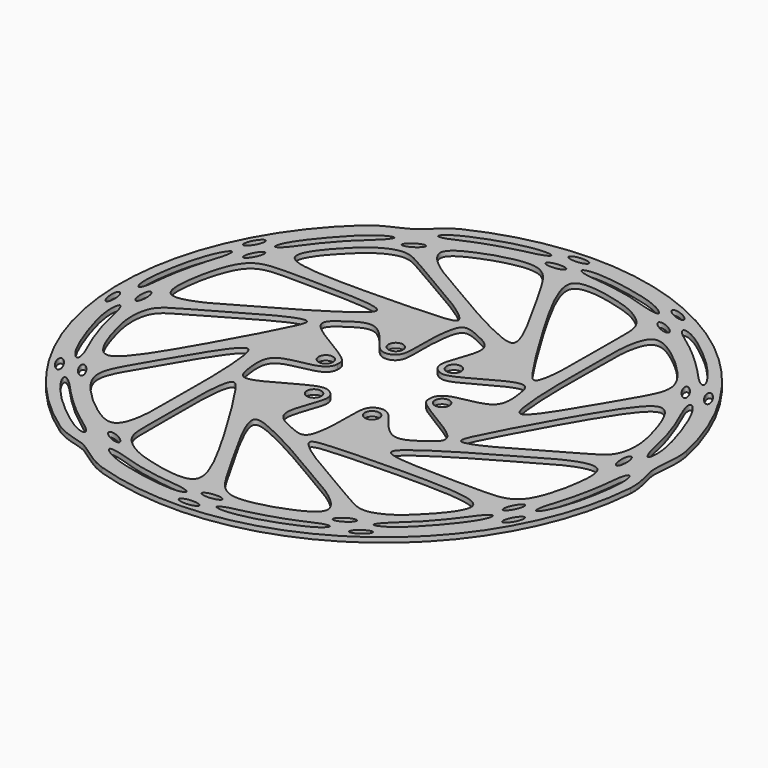
from build123d import *

# Parameters (mm, degrees)
F0_R             = 100
F1_DEPTH         = 1.85
F2_R             = 2.743128254
F3_DEPTH         = 1.851
F3_COPIES_COUNT  = 6
F7_DEPTH         = 1.8510001
F7_COPIES_COUNT  = 3
F10_DEPTH        = 1.8510001
F10_COPIES_COUNT = 2


# Not quite as in the source:
# - a pattern or mirror of a feature is missing from the dataset's text; its kind, count and spacing are read off the source's solid


with BuildPart() as f1:
    # F0 (on Top) → F1 (new body)
    with BuildSketch(Plane.XY):
        Circle(F0_R)
    extrude(amount=F1_DEPTH)

    # F2 (on Top) → F3 (cut, through all)
    with BuildSketch(Plane.XY):
        with BuildLine():
            add(Edge.make_bspline(
                [(-19.3818919361, 84.770321846), (-15.8888721091, 85.5119795187), (-7.6996501995, 86.6691177995), (-1.2711069947, 76.0041983595), (2.7590544213, 68.8211609673), (14.2848097306, 48.826735121), (15.6555298575, 41.0029385401), (4.0306774131, 45.832846657), (-11.3442409562, 54.3632933665), (-25.1795732316, 62.8245536026), (-31.577920473, 66.1201997026), (-42.6321499163, 75.6247304734), (-28.620182769, 82.2286800508), (-22.8365351394, 84.0368125145), (-19.3818919361, 84.770321846)],
                knots=[0, 0, 0, 0, 0.0806437638, 0.1605805509, 0.2363933489, 0.3555478125, 0.4090968647, 0.4834244698, 0.5923152663, 0.6895970753, 0.7594857624, 0.8380620694, 0.9202422418, 1, 1, 1, 1], degree=3))
        make_face()
        with BuildLine():
            add(Edge.make_bspline(
                [(4.0786904283, 83.0234959722), (4.8408661308, 85.0940211581), (10.9812602111, 85.7206275438), (19.6535574621, 83.7725691497), (28.668941965, 81.3282055643), (36.9257742239, 75.2245847174), (36.9680314736, 65.9345839836), (36.8019909238, 45.080539991), (36.8744568041, 36.732354482), (35.337710167, 25.8934041706), (29.5967546476, 32.9556866993), (17.5290674718, 52.9370163353), (11.4660357229, 63.1418800906), (2.7822748423, 79.5016556493), (4.0786904283, 83.0234959722)],
                knots=[0, 0, 0, 0, 0.0635478904, 0.1391827355, 0.2151092654, 0.2891479476, 0.3630886814, 0.4747583724, 0.5526009533, 0.6195279395, 0.6767941119, 0.7963800874, 0.8919088141, 1, 1, 1, 1], degree=3))
        make_face()
        with Locations((11.2100625411, 19.0960504115)):
            Circle(F2_R)
        with BuildLine():
            add(Edge.make_bspline(
                [(1.3292516815, 91.8782353401), (1.2925002073, 92.3354583441), (4.9372757242, 93.8495882438), (20.9611120073, 91.4975725839), (33.039082784, 87.9708444738), (37.8500908983, 83.7397445096), (31.1774053281, 84.75909445), (24.9839859282, 87.3881882236), (11.578213695, 89.906480861), (4.1885603815, 90.1973514145), (1.3641017607, 91.4446674832), (1.3292516815, 91.8782353401)],
                knots=[0, 0, 0, 0, 0.069104069, 0.2382448936, 0.392001905, 0.4676969543, 0.5517462119, 0.6661598603, 0.8182820791, 0.9344711381, 1, 1, 1, 1], degree=3))
        make_face()
        with BuildLine():
            add(Edge.make_bspline(
                [(-2.7077326085, 89.5969420671), (-2.8745052619, 91.7024450684), (-8.261381892, 90.2164050531), (-13.6482585222, 88.7303650379), (-8.0946092387, 88.1109020519), (-2.5409599552, 87.4914390659), (-2.7077326085, 89.5969420671)],
                knots=[0, 0, 0, 2.0943951024, 2.0943951024, 4.1887902048, 4.1887902048, 6.2831853072, 6.2831853072, 6.2831853072], degree=2, weights=[1, 0.5, 1, 0.5, 1, 0.5, 1]))
        make_face()
        with BuildLine():
            add(Edge.make_bspline(
                [(0.2530701458, 96.746198833), (0.1434808405, 98.981842031), (-5.3261488772, 97.5932179043), (-10.7957785949, 96.2045937777), (-5.2165595719, 95.3575747063), (0.3626594512, 94.510555635), (0.2530701458, 96.746198833)],
                knots=[0, 0, 0, 2.0943951024, 2.0943951024, 4.1887902048, 4.1887902048, 6.2831853072, 6.2831853072, 6.2831853072], degree=2, weights=[1, 0.5, 1, 0.5, 1, 0.5, 1]))
        make_face()
        with BuildLine():
            add(Edge.make_bspline(
                [(-45.5902777612, 82.5898870826), (-45.8140727222, 82.9738085349), (-43.585623242, 85.7456500755), (-33.1460813636, 90.1844826755), (-22.9095160971, 93.5693996934), (-13.6129666728, 94.789503836), (-10.8334910775, 93.6639122431), (-14.5180403097, 91.7933261946), (-21.5013009013, 90.6303087594), (-35.2407786326, 86.3505494796), (-42.3849200633, 82.5115902384), (-45.3821119555, 82.2327775296), (-45.5902777612, 82.5898870826)],
                knots=[0, 0, 0, 0, 0.065019585, 0.198537651, 0.3338114005, 0.4526335757, 0.5018406824, 0.5658849331, 0.6740049001, 0.8245613986, 0.9395211838, 1, 1, 1, 1], degree=3))
        make_face()
    f3 = extrude(amount=F3_DEPTH, mode=Mode.SUBTRACT)

    # F3_copies: F3 ×6 about axis
    f3_copies_axis = Axis((0, 0, 0), (0, 0, 1))
    for i in range(1, F3_COPIES_COUNT):
        add(f3.rotate(f3_copies_axis, i * 360 / F3_COPIES_COUNT), mode=Mode.SUBTRACT)

    # F5 (on Top) → F7 (cut, through all)
    with BuildSketch(Plane.XY):
        with BuildLine():
            add(Edge.make_bspline(
                [(44.7057709098, 85.9585851431), (45.5545956472, 87.8521204143), (40.2434163829, 89.0959687605), (34.9322371185, 90.3398171067), (39.3945916454, 87.2024334893), (43.8569461723, 84.0650498719), (44.7057709098, 85.9585851431)],
                knots=[0, 0, 0, 2.0943951024, 2.0943951024, 4.1887902048, 4.1887902048, 6.2831853072, 6.2831853072, 6.2831853072], degree=2, weights=[1, 0.5, 1, 0.5, 1, 0.5, 1]))
        make_face()
        with BuildLine():
            add(Edge.make_bspline(
                [(46.2925173342, 76.8029242754), (47.3216432051, 78.7262145228), (42.0045682647, 80.3343268011), (36.6874933243, 81.9424390793), (40.9754423938, 78.4110365536), (45.2633914634, 74.879634028), (46.2925173342, 76.8029242754)],
                knots=[0, 0, 0, 2.0943951024, 2.0943951024, 4.1887902048, 4.1887902048, 6.2831853072, 6.2831853072, 6.2831853072], degree=2, weights=[1, 0.5, 1, 0.5, 1, 0.5, 1]))
        make_face()
        with BuildLine():
            add(Edge.make_bspline(
                [(-44.3659611046, 75.4196792841), (-45.4973806998, 77.214342523), (-49.5406950544, 73.4113179984), (-53.584009409, 69.6082934737), (-48.4092754592, 71.6166547595), (-43.2345415094, 73.6250160452), (-44.3659611046, 75.4196792841)],
                knots=[0, 0, 0, 2.0943951024, 2.0943951024, 4.1887902048, 4.1887902048, 6.2831853072, 6.2831853072, 6.2831853072], degree=2, weights=[1, 0.5, 1, 0.5, 1, 0.5, 1]))
        make_face()
        with BuildLine():
            ThreePointArc((99.6824280645, -7.9632615906), (99.7801919642, 6.6267104655), (97.7538666441, 21.0756152016))
            add(Edge.make_bspline(
                [(97.7538666441, 21.0756152016), (99.0152444039, 13.9993348283), (95.754510368, 5.1865162185), (99.9780440485, -2.0954016886), (99.6824280645, -7.9632615906)],
                knots=[0, 0, 0, 0, 0.5215356481, 1, 1, 1, 1], degree=3))
        make_face()
    f7 = extrude(amount=F7_DEPTH, mode=Mode.SUBTRACT)

    # F7_copies: F7 ×3 about axis
    f7_copies_axis = Axis((0, 0, 0), (0, 0, 1))
    for i in range(1, F7_COPIES_COUNT):
        add(f7.rotate(f7_copies_axis, i * 360 / F7_COPIES_COUNT), mode=Mode.SUBTRACT)

    # F8 (on Top) → F10 (cut, through all)
    with BuildSketch(Plane.XY):
        with BuildLine():
            add(Edge.make_bspline(
                [(-17.5606684038, 0), (-17.5606684038, 1.2998864508), (-17.2074510032, 3.8889565681), (-34.449153164, 12.5684504715), (-39.0439728452, 18.4831422726), (-32.6302785782, 23.066897504), (-24.7304969857, 28.0832041862), (-17.4208398269, 20.0646092064), (-12.9792845116, 13.2889788045), (-5.8501060437, 15.2620458951), (-6.2247287127, 24.4663670609), (-5.8417294967, 36.461497552), (-3.4888554678, 43.1450124033), (3.6529640524, 39.9447930175), (13.5957501242, 35.3949556325), (4.4850047832, 19.4249977015), (8.2201400332, 14.902367155), (13.6783342254, 12.9988158846), (34.797754889, 28.4572435269), (36.4856634042, 18.0279806875), (37.7083841418, 6.0979547197), (20.2202463654, 5.9816753456), (17.5606684038, 1.6842670971), (17.5606684038, 0)],
                knots=[0, 0, 0, 0, 0.0295655241, 0.1002359319, 0.1402627169, 0.1819917002, 0.2290112946, 0.2794797726, 0.3249086986, 0.3613438617, 0.4086075502, 0.4673128145, 0.5047300957, 0.5465400616, 0.5948481409, 0.6587742082, 0.6933540172, 0.7304882104, 0.8069708011, 0.8482147969, 0.8992901591, 0.9618023593, 1, 1, 1, 1], degree=3))
            Line((-17.5606684038, 0), (17.5606684038, 0))
        make_face()
    f10 = extrude(amount=F10_DEPTH, mode=Mode.SUBTRACT)

    # F10_copies: F10 ×2 about axis
    f10_copies_axis = Axis((0, 0, 0), (0, 0, 1))
    for i in range(1, F10_COPIES_COUNT):
        add(f10.rotate(f10_copies_axis, i * 360 / F10_COPIES_COUNT), mode=Mode.SUBTRACT)


solid = f1.part
